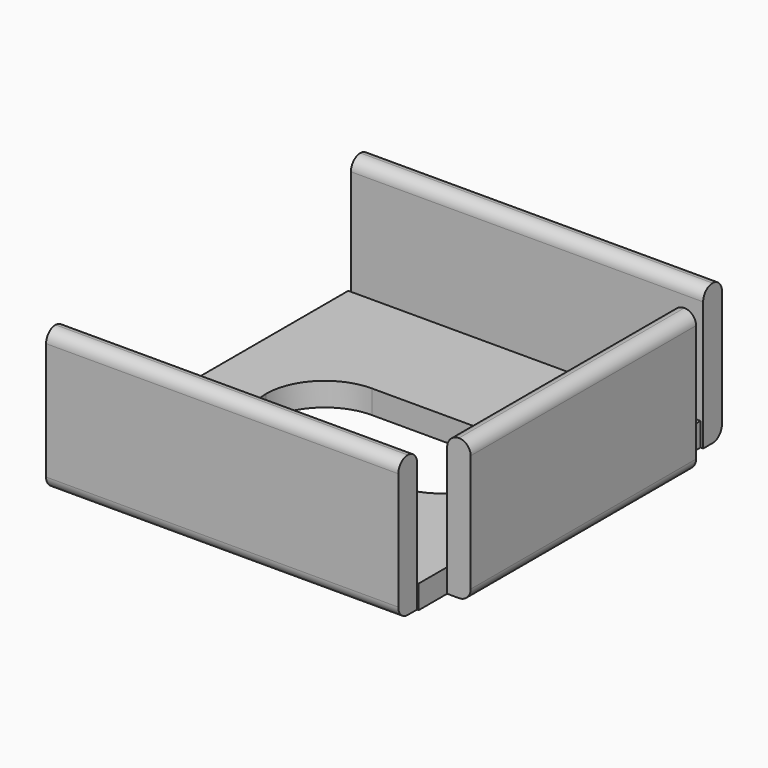
from build123d import *

# Parameters (mm, degrees)
F9_W      = 12
F9_H      = 6
F10_DEPTH = 1
F8_W      = 15
F8_H      = 6
F11_DEPTH = 1
F7_W      = 15
F7_H      = 6
F12_DEPTH = 1
F0_W      = 15
F0_H      = 15
F13_DEPTH = 1
F14_R     = 0.5
F15_R     = 0.49999
F15_2_R   = 0.49999
F16_R     = 0.49999
F16_2_R   = 0.49999
F17_DEPTH = 1


# Not quite as in the source:
# - a fillet or chamfer is up to 0.001 mm smaller than in the source, because OpenCascade refuses the exact size


with BuildPart() as f10:
    # F9 (on plane+point) → F10 (new body)
    with BuildSketch(Plane.YZ.offset(7.5)):
        with Locations((0.0150063767, 3)):
            Rectangle(F9_W, F9_H)
    extrude(amount=F10_DEPTH)

    # F14
    f14_edges = [f10.edges().sort_by_distance(p)[0] for p in [
        (8.5, 0.015006, 6),
    ]]
    fillet(f14_edges, radius=F14_R)

    # F15 (radius 0.5 in the source; OpenCascade refuses exactly that, so slightly less here)
    f15_edges = [f10.edges().sort_by_distance(p)[0] for p in [
        (7.5, 0.015006, 6),
        (8.5, 0.015006, 0),
    ]]
    fillet(f15_edges, radius=F15_R)

    # F0 (on Top) → F17 (cut)
    with BuildSketch(Plane.XY):
        with BuildLine():
            Line((2.5, 2.5), (-2.5, 2.5))
            ThreePointArc((-2.5, 2.5), (-4.267766953, 1.767766953), (-5, 0))
            ThreePointArc((-5, 0), (-4.267766953, -1.767766953), (-2.5, -2.5))
            Line((-2.5, -2.5), (2.5, -2.5))
            ThreePointArc((2.5, -2.5), (4.267766953, -1.767766953), (5, 0))
            ThreePointArc((5, 0), (4.267766953, 1.767766953), (2.5, 2.5))
        make_face()
    extrude(amount=F17_DEPTH, mode=Mode.SUBTRACT)


with BuildPart() as f11:
    # F8 (on plane+point) → F11 (new body)
    with BuildSketch(Plane.XZ.offset(-7.5)):
        with Locations((0.1134890686, 3)):
            Rectangle(F8_W, F8_H)
    extrude(amount=-F11_DEPTH)

    # F0 (on Top) → F13 (join)
    with BuildSketch(Plane.XY):
        Rectangle(F0_W, F0_H)
        with BuildLine():
            ThreePointArc((-5, 0), (-4.267766953, 1.767766953), (-2.5, 2.5))
            Line((-2.5, 2.5), (2.5, 2.5))
            ThreePointArc((2.5, 2.5), (4.267766953, 1.767766953), (5, 0))
            ThreePointArc((5, 0), (4.267766953, -1.767766953), (2.5, -2.5))
            Line((2.5, -2.5), (-2.5, -2.5))
            ThreePointArc((-2.5, -2.5), (-4.267766953, -1.767766953), (-5, 0))
        make_face(mode=Mode.SUBTRACT)
    extrude(amount=F13_DEPTH)

    # F16#2 (radius 0.5 in the source; OpenCascade refuses exactly that, so slightly less here)
    f16_2_edges = [f11.edges().sort_by_distance(p)[0] for p in [
        (0.113489, 8.5, 0),
        (0.113489, 8.5, 6),
        (0.113489, 7.5, 6),
    ]]
    fillet(f16_2_edges, radius=F16_2_R)


with BuildPart() as f12:
    # F7 (on plane+point) → F12 (new body)
    with BuildSketch(Plane.XZ.offset(7.5)):
        with Locations((-0.0702422911, 3)):
            Rectangle(F7_W, F7_H)
    extrude(amount=F12_DEPTH)

    # F15#2 (radius 0.5 in the source; OpenCascade refuses exactly that, so slightly less here)
    f15_2_edges = [f12.edges().sort_by_distance(p)[0] for p in [
        (-0.070242, -8.5, 6),
        (-0.070242, -7.5, 6),
    ]]
    fillet(f15_2_edges, radius=F15_2_R)

    # F16 (radius 0.5 in the source; OpenCascade refuses exactly that, so slightly less here)
    f16_edges = [f12.edges().sort_by_distance(p)[0] for p in [
        (-0.070242, -8.5, 0),
    ]]
    fillet(f16_edges, radius=F16_R)


solid = Compound([f10.part, f11.part, f12.part])
